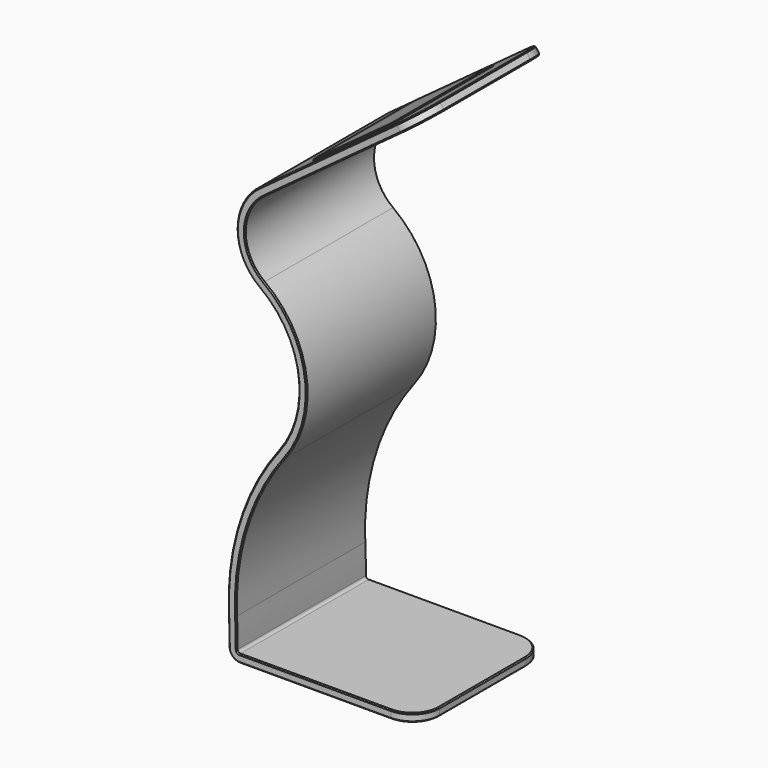
from build123d import *

# Parameters (mm, degrees)
F1_DEPTH = 150
F2_W     = 150
F2_H     = 200
F3_DEPTH = 8
F4_DEPTH = 2
F5_DEPTH = 2
F6_SIZE  = 0.5
F7_R     = 50
F8_SIZE  = 2


with BuildPart() as f1:
    # F0 (on Front) → F1 (new body, symmetric)
    with BuildSketch(Plane.XZ):
        with BuildLine():
            ThreePointArc((0, 20), (5.8578643763, 5.8578643763), (20, 0))
            Line((20, 0), (349.2813145287, 0))
            Line((349.2813145287, 0), (349.2813145287, 15))
            Line((349.2813145287, 15), (20, 15))
            ThreePointArc((20, 15), (16.4644660941, 16.4644660941), (15, 20))
            ThreePointArc((15, 20), (14.6952395355, 46.9639715527), (13.7811138505, 73.9141666367))
            ThreePointArc((13.7811138505, 73.9141666367), (33.5445295719, 224.9539574175), (103.9868612693, 360.0150136294))
            ThreePointArc((103.9868612693, 360.0150136294), (142.242823173, 505.2528295697), (65.0920324936, 634.1143726997))
            ThreePointArc((65.0920324936, 634.1143726997), (29.9146009128, 703.5392819502), (65.0920324936, 772.9641912008))
            Line((65.0920324936, 772.9641912008), (358.1525547883, 987.9045009919))
            Line((358.1525547883, 987.9045009919), (349.2813145287, 1000))
            Line((349.2813145287, 1000), (56.2207922339, 785.0596902089))
            ThreePointArc((56.2207922339, 785.0596902089), (14.9146009128, 703.5392819502), (56.2207922339, 622.0188736916))
            ThreePointArc((56.2207922339, 622.0188736916), (127.3915982157, 503.1454337196), (92.1008692639, 369.1650515553))
            ThreePointArc((92.1008692639, 369.1650515553), (19.2387537556, 229.4644760457), (-1.2035604669, 73.236276084))
            ThreePointArc((-1.2035604669, 73.236276084), (-0.3009285544, 46.624939667), (0, 20))
        make_face()
    extrude(amount=F1_DEPTH, both=True)

    # F2 (on face) → F3 (cut)
    with BuildSketch(Plane(origin=(-354.7289831539, 0, 483.6554910394), x_dir=(0.8063666005, 0, 0.5914160173), z_dir=(-0.5914160173, 0, 0.8063666005))):
        with BuildLine():
            Line((598.8481239922, 108), (598.8481239922, -108))
            ThreePointArc((598.8481239922, -108), (602.3628426179, -116.4852813742), (610.8481239922, -120))
            Line((610.8481239922, -120), (771.8481239922, -120))
            ThreePointArc((771.8481239922, -120), (780.3334053664, -116.4852813742), (783.8481239922, -108))
            Line((783.8481239922, -108), (783.8481239922, 108))
            ThreePointArc((783.8481239922, 108), (780.3334053664, 116.4852813742), (771.8481239922, 120))
            Line((771.8481239922, 120), (610.8481239922, 120))
            ThreePointArc((610.8481239922, 120), (602.3628426179, 116.4852813742), (598.8481239922, 108))
        make_face()
        with Locations((691.3481239922, 0)):
            Rectangle(F2_W, F2_H, mode=Mode.SUBTRACT)
        with Locations((691.3481239922, 0)):
            Rectangle(F2_W, F2_H)
    extrude(amount=-F3_DEPTH, mode=Mode.SUBTRACT)

    # F7
    f7_edges = [f1.edges().sort_by_distance(p)[0] for p in [
        (353.716935, -150, 993.95225),
        (353.716935, 150, 993.95225),
        (349.281315, -150, 7.5),
        (349.281315, 150, 7.5),
    ]]
    fillet(f7_edges, radius=F7_R)

    # F8
    f8_edges = [f1.edges().sort_by_distance(p)[0] for p in [
        (349.281315, 0, 1000),
        (202.751053, -120, 892.529845),
        (358.152555, 0, 987.904501),
    ]]
    chamfer(f8_edges, length=F8_SIZE)


with BuildPart() as f4:
    # F2 (on face) → F4 (new body)
    with BuildSketch(Plane(origin=(-354.7289831539, 0, 483.6554910394), x_dir=(0.8063666005, 0, 0.5914160173), z_dir=(-0.5914160173, 0, 0.8063666005))):
        with BuildLine():
            Line((598.8481239922, 108), (598.8481239922, -108))
            ThreePointArc((598.8481239922, -108), (602.3628426179, -116.4852813742), (610.8481239922, -120))
            Line((610.8481239922, -120), (771.8481239922, -120))
            ThreePointArc((771.8481239922, -120), (780.3334053664, -116.4852813742), (783.8481239922, -108))
            Line((783.8481239922, -108), (783.8481239922, 108))
            ThreePointArc((783.8481239922, 108), (780.3334053664, 116.4852813742), (771.8481239922, 120))
            Line((771.8481239922, 120), (610.8481239922, 120))
            ThreePointArc((610.8481239922, 120), (602.3628426179, 116.4852813742), (598.8481239922, 108))
        make_face()
        with Locations((691.3481239922, 0)):
            Rectangle(F2_W, F2_H, mode=Mode.SUBTRACT)
    extrude(amount=F4_DEPTH)

    # F6
    f6_edges = [f4.edges().sort_by_distance(p)[0] for p in [
        (201.568221, -120, 894.142578),
    ]]
    chamfer(f6_edges, length=F6_SIZE)


with BuildPart() as f5:
    # F2 (on face) → F5 (new body)
    with BuildSketch(Plane(origin=(-354.7289831539, 0, 483.6554910394), x_dir=(0.8063666005, 0, 0.5914160173), z_dir=(-0.5914160173, 0, 0.8063666005))):
        with Locations((691.3481239922, 0)):
            Rectangle(F2_W, F2_H)
    extrude(amount=F5_DEPTH)


solid = Compound([f1.part, f4.part, f5.part])
